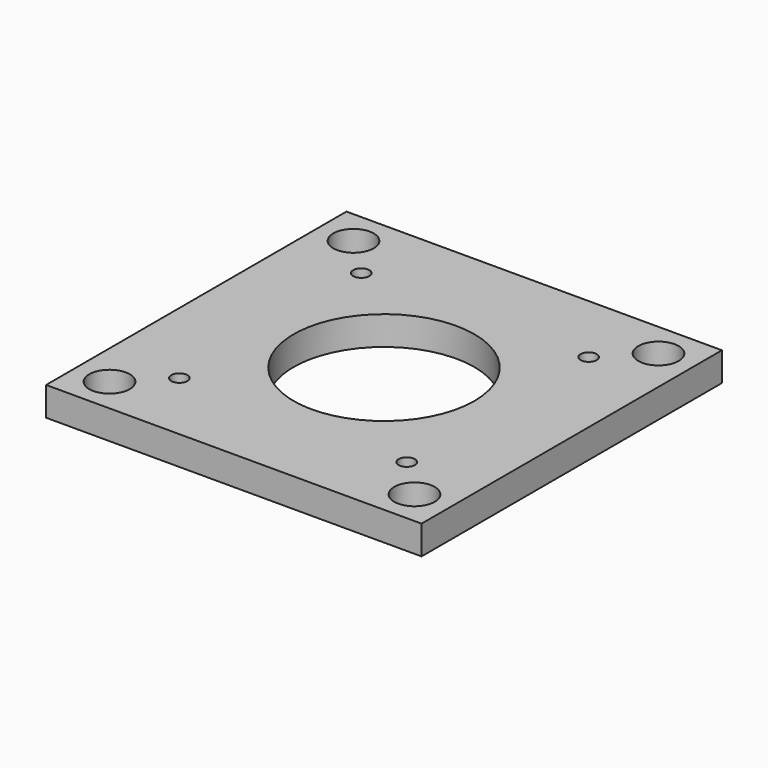
from build123d import *

# Parameters (mm, degrees)
F0_W     = 82.55
F0_H     = 82.55
F0_R     = 4.445
F0_R_2   = 1.778
F0_R_3   = 19.8755
F1_DEPTH = 6.35


# Not quite as in the source:
# - a length typed as a fraction of an inch, garbled in the dataset ("3 / 203.2 mm" for 3/8 in), is restored


with BuildPart() as f1:
    # F0 (on Top) → F1 (new body)
    with BuildSketch(Plane.XY):
        Rectangle(F0_W, F0_H)
        with Locations((-33.528, -33.528)):
            Circle(F0_R, mode=Mode.SUBTRACT)
        with Locations((-24.9936, -24.9936)):
            Circle(F0_R_2, mode=Mode.SUBTRACT)
        with Locations((33.528, -33.528)):
            Circle(F0_R, mode=Mode.SUBTRACT)
        with Locations((24.9936, -24.9936)):
            Circle(F0_R_2, mode=Mode.SUBTRACT)
        with Locations((-24.9936, 24.9936)):
            Circle(F0_R_2, mode=Mode.SUBTRACT)
        with Locations((-33.528, 33.528)):
            Circle(F0_R, mode=Mode.SUBTRACT)
        Circle(F0_R_3, mode=Mode.SUBTRACT)
        with Locations((24.9936, 24.9936)):
            Circle(F0_R_2, mode=Mode.SUBTRACT)
        with Locations((33.528, 33.528)):
            Circle(F0_R, mode=Mode.SUBTRACT)
    extrude(amount=F1_DEPTH)


solid = f1.part
